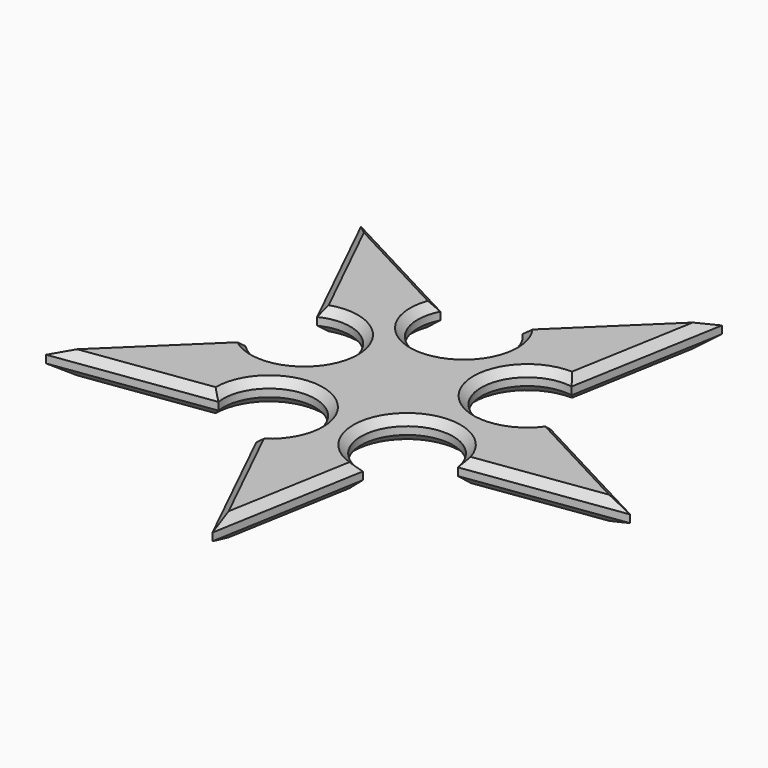
from build123d import *

# Parameters (mm, degrees)
F1_DEPTH = 4.7625
F2_R     = 9.525
F3_DEPTH = 4.7635
F4_SIZE  = 1.5875


# Not quite as in the source:
# - a feature of the source that left no trace in its solid (it failed there, or was rolled back) is left out


with BuildPart() as f1:
    # F0 (on Top) → F1 (new body)
    with BuildSketch(Plane.XY):
        Polygon((-3.074264621, 21.805118867), (-40.0660246394, 41.4531760826), (-21.6879004002, 3.8143528936), (-51.8053957451, -25.295317935), (-10.3295949709, -19.4477191337), (8.0485292683, -57.0865423226), (15.3038596181, -15.8337043219), (56.7796603923, -9.9861055206), (19.787900374, 9.6619516949), (27.0432307238, 50.9147896956), align=None)
    extrude(amount=F1_DEPTH)

    # F2 (on Top) → F3 (cut, through all)
    with BuildSketch(Plane.XY):
        with Locations((15.3038596181, -15.8337043219)):
            Circle(F2_R)
        with Locations((-10.3295949709, -19.4477191337)):
            Circle(F2_R)
        with Locations((-21.6879004002, 3.8143528936)):
            Circle(F2_R)
        with Locations((-3.074264621, 21.805118867)):
            Circle(F2_R)
        with Locations((19.787900374, 9.6619516949)):
            Circle(F2_R)
    extrude(amount=F3_DEPTH, mode=Mode.SUBTRACT)

    # F4
    f4_edges = [f1.edges().sort_by_distance(p)[0] for p in [
        (24.240507, 34.97888, 4.7625),
        (15.408887, 39.669767, 4.7625),
        (-1.744503, 12.373398, 4.7625),
        (-25.776163, 33.863161, 4.7625),
        (-32.966583, 26.913355, 4.7625),
        (-12.306882, 2.164469, 4.7625),
        (-40.171052, -14.050296, 4.7625),
        (-35.783356, -23.036399, 4.7625),
        (-5.861568, -11.035682, 4.7625),
        (0.949087, -42.546721, 4.7625),
        (10.851253, -41.150633, 4.7625),
        (8.684234, -8.984896, 4.7625),
        (40.75762, -12.245024, 4.7625),
        (42.489799, -2.39609, 4.7625),
        (11.22872, 5.482711, 4.7625),
        (24.240507, 34.97888, 0),
        (15.408887, 39.669767, 0),
        (-1.744503, 12.373398, 0),
        (-25.776163, 33.863161, 0),
        (-32.966583, 26.913355, 0),
        (-12.306882, 2.164469, 0),
        (-40.171052, -14.050296, 0),
        (-35.783356, -23.036399, 0),
        (-5.861568, -11.035682, 0),
        (0.949087, -42.546721, 0),
        (10.851253, -41.150633, 0),
        (8.684234, -8.984896, 0),
        (40.75762, -12.245024, 0),
        (42.489799, -2.39609, 0),
        (11.22872, 5.482711, 0),
    ]]
    chamfer(f4_edges, length=F4_SIZE)


solid = f1.part
